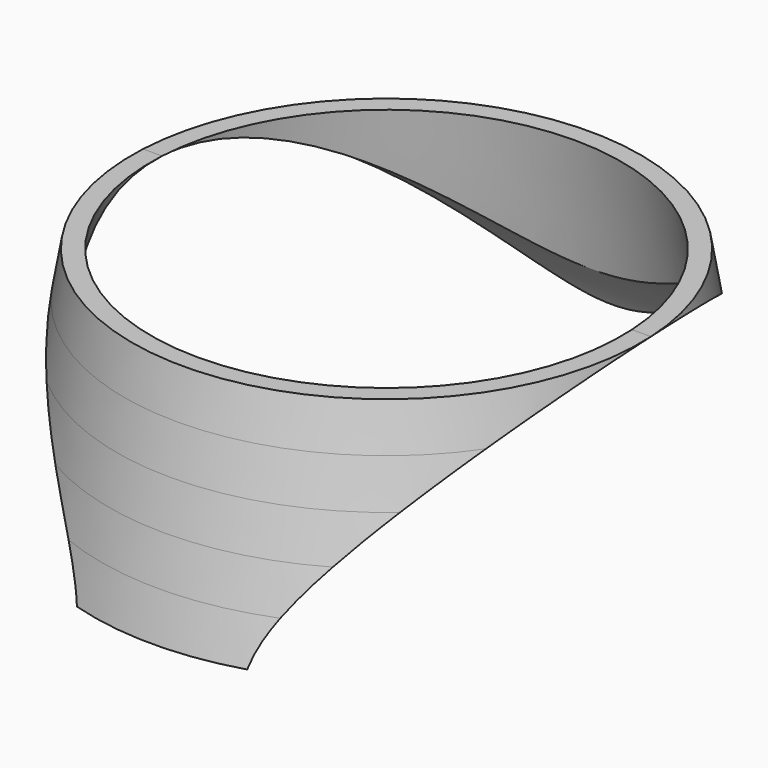
from build123d import *
from build123d import SkipClean  # not in build123d's __all__

# Parameters (mm, degrees)
F2_R     = 4050
F3_DEPTH = 5000
F7_W     = 10000
F7_H     = 0.001
F8_DEPTH = 5000


with BuildPart() as f1:
    # F0 (on Right) → F1 (revolve)
    with BuildSketch(Plane.YZ):
        Polygon((-3666.4068231672, -1517.7600373064), (-3146.4068231672, 1538.315877981), (-3400, 1538.315877981), (-3920, -1517.7600373064), align=None)
    revolve(axis=Axis((0, 0, 521.2879776955), (0, 0, 1)))

    # F2 (on Right) → F3 (cut, symmetric)
    with BuildSketch(Plane.YZ):
        with Locations((175, -2511.684122019)):
            Circle(F2_R)
    with SkipClean():  # cleaning this boolean's faces spoils the solid; the shape is the same uncleaned
        extrude(amount=F3_DEPTH, both=True, mode=Mode.SUBTRACT)

    # F7 (on Right) → F8 (cut, symmetric)
    with BuildSketch(Plane.YZ):
        with Locations((-5000, 927.115377981)):
            Rectangle(F7_W, F7_H)
        with Locations((-5000, 313.915377981)):
            Rectangle(F7_W, F7_H)
        with Locations((-5000, -297.284622019)):
            Rectangle(F7_W, F7_H)
        with Locations((-5000, -908.484622019)):
            Rectangle(F7_W, F7_H)
    extrude(amount=F8_DEPTH, both=True, mode=Mode.SUBTRACT)


solid = f1.part
